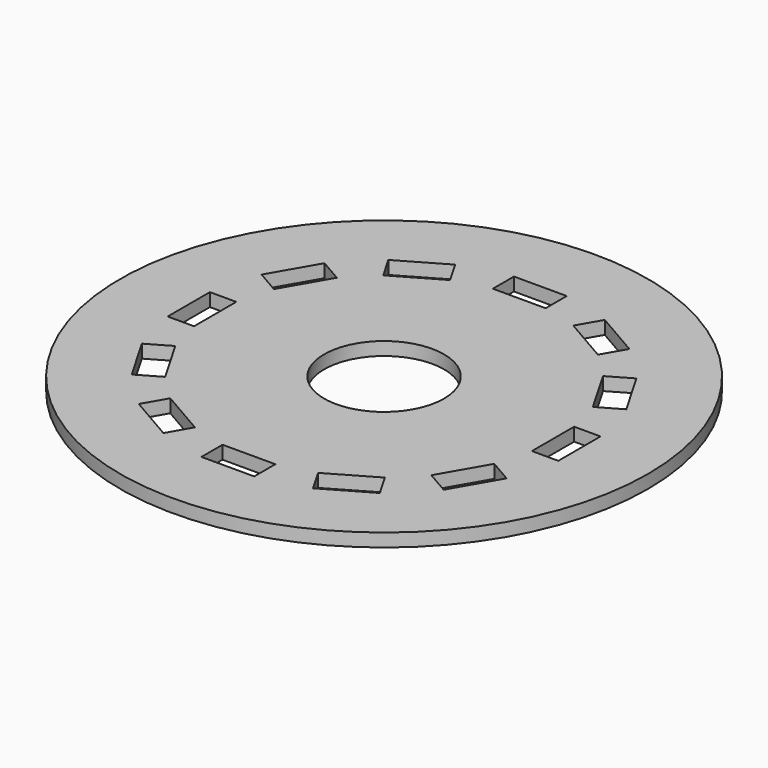
from build123d import *

# Parameters (mm, degrees)
F0_R            = 63.5
F0_R_2          = 14.4272
F1_DEPTH        = 3.175
F2_W            = 12.7
F2_H            = 6.35
F3_DEPTH        = 3.176
F3_COPIES_COUNT = 12
F4_R            = 2.4892
F5_DEPTH        = 182


# Not quite as in the source:
# - an extrude ends at something that could not be found from the text; its depth is read off the source's solid
# - a pattern or mirror of a feature is missing from the dataset's text; its kind, count and spacing are read off the source's solid


with BuildPart() as f1:
    # F0 (on Top) → F1 (new body)
    with BuildSketch(Plane.XY):
        Circle(F0_R)
        Circle(F0_R_2, mode=Mode.SUBTRACT)
    extrude(amount=F1_DEPTH)

    # F2 (on face) → F3 (cut, through all)
    with BuildSketch(Plane.XY.offset(3.175)):
        with Locations((0, 43.815)):
            Rectangle(F2_W, F2_H)
    f3 = extrude(amount=-F3_DEPTH, mode=Mode.SUBTRACT)

    # F3_copies: F3 ×12 about axis
    f3_copies_axis = Axis((0, 0, 0), (0, 0, 1))
    for i in range(1, F3_COPIES_COUNT):
        add(f3.rotate(f3_copies_axis, i * 360 / F3_COPIES_COUNT), mode=Mode.SUBTRACT)

    # F4 (on Top) → F5 (cut, through all)
    with BuildSketch(Plane.XY):
        with Locations((0, 23.8125)):
            Circle(F4_R)
    extrude(amount=-F5_DEPTH, mode=Mode.SUBTRACT)


solid = f1.part
